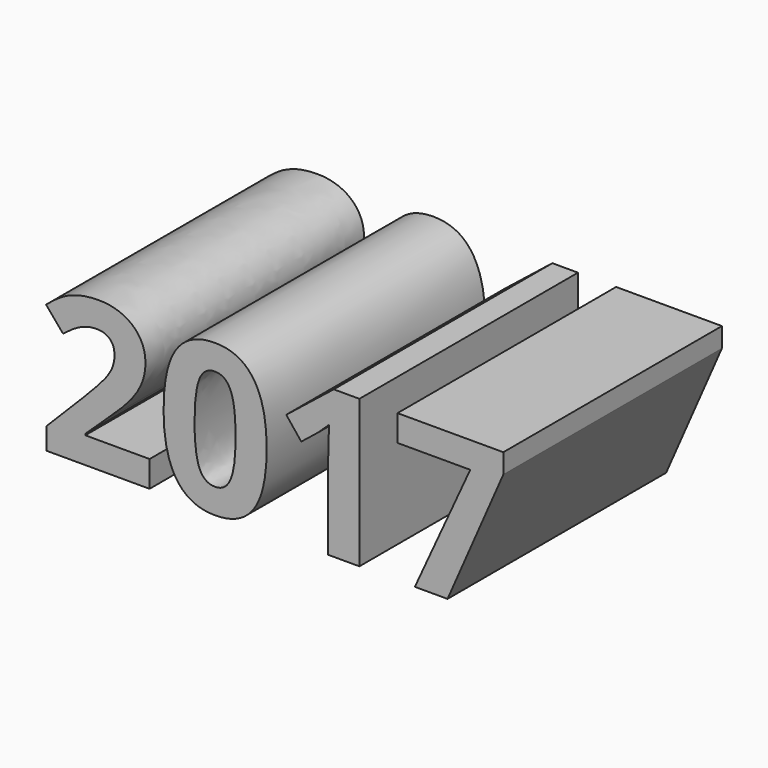
from build123d import *

# Parameters (mm, degrees)
F0_TEXT_SIZE = 19.2044884898
F1_DEPTH     = 25.4


# Not quite as in the source:
# - Text() gives the source's letters only with a copy of the font that has no kerning and outlines rounded to 1/6400 em; it was checked with that copy


with BuildPart() as f1:
    # F0 (on Front) → F1 (new body)
    with BuildSketch(Plane.XZ):
        with Locations((-44.4823964644, 0)):
            Text('2017', F0_TEXT_SIZE, font='Open Sans', font_style=FontStyle.BOLD, text_align=(TextAlign.LEFT, TextAlign.BOTTOM))
    extrude(amount=F1_DEPTH)


solid = f1.part
